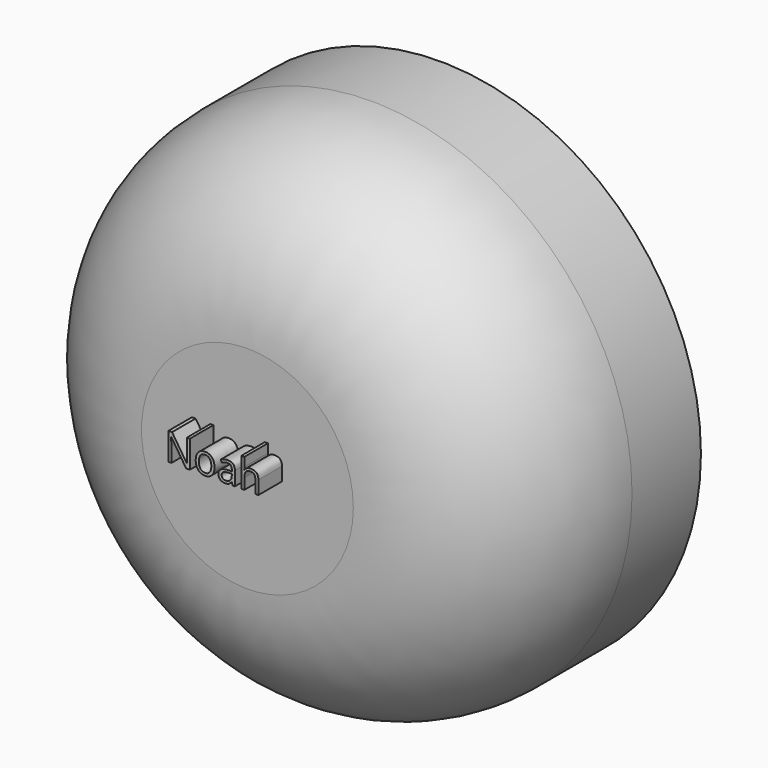
from build123d import *

# Parameters (mm, degrees)
F0_R         = 38.2060265377
F1_DEPTH     = 35.306
F2_R         = 22.6887790592
F3_T         = -2.54
F4_TEXT_SIZE = 5.6092808437
F5_DEPTH     = 39.624


# Not quite as in the source:
# - Text() gives the source's letters only with a copy of the font that has no kerning and outlines rounded to 1/6400 em; it was checked with that copy


with BuildPart() as f1:
    # F0 (on Front) → F1 (new body)
    with BuildSketch(Plane.XZ):
        Circle(F0_R)
    extrude(amount=F1_DEPTH)

    # F2
    f2_edges = [f1.edges().sort_by_distance(p)[0] for p in [
        (-38.206027, -35.306, 0),
    ]]
    fillet(f2_edges, radius=F2_R)

    # F3
    f3_openings = [f1.faces().sort_by_distance(p)[0] for p in [
        (0, 0, 0),
    ]]
    offset(amount=F3_T, openings=f3_openings)

    # F4 (on Front) → F5 (join)
    with BuildSketch(Plane.XZ):
        with Locations((-8.6648818105, 0)):
            Text('Noah', F4_TEXT_SIZE, font='Open Sans', text_align=(TextAlign.LEFT, TextAlign.BOTTOM))
    extrude(amount=F5_DEPTH)


solid = f1.part
